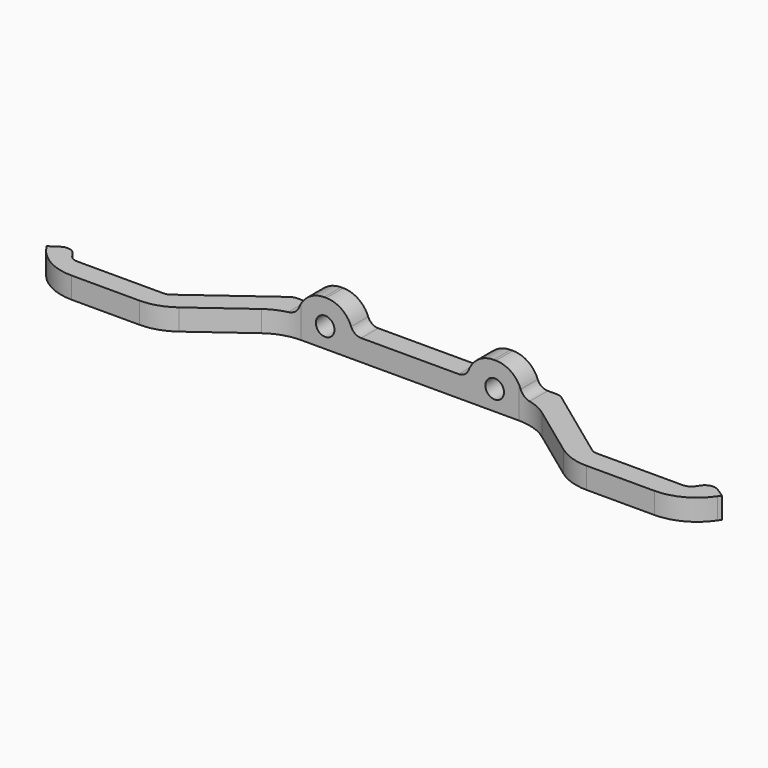
from build123d import *

# Parameters (mm, degrees)
F1_DEPTH    = 4
F2_W        = 9.5
F2_H        = 8.5
F3_DEPTH    = 4
F4_R        = 1.75
F5_DEPTH    = 154
F6_R        = 10
F7_R        = 2
F8_R        = 2
F9_T1_DEPTH = 26.6944612474
F9_T3_DEPTH = 26.6917420766


# Not quite as in the source:
# - a fillet or chamfer that OpenCascade refuses, or shapes differently, is made with other operations: its cross-section is extruded or revolved along the edge and cut away or added
# - an extrude ends at something that could not be found from the text; its depth is read off the source's solid


with BuildPart() as f1:
    # F0 (on Top) → F1 (new body)
    with BuildSketch(Plane.XY):
        Polygon((-82.859264966, -11), (-85, -7.7888974491), (-88.3282011774, -10.007698234), (-85, -15), (-63.6905180954, -15), (-48.6905180954, -4), (-1.3094819046, -4), (13.6905180954, -15), (35, -15), (38.3282011774, -10.007698234), (35, -7.7888974491), (32.859264966, -11), (15, -11), (0, 0), (-50, 0), (-65, -11), align=None)
    extrude(amount=F1_DEPTH)

    # F2 (on face) → F3 (join, through all)
    with BuildSketch(Plane(origin=(0, 0, 0), x_dir=(-1, 0, 0), z_dir=(0, 1, 0))):
        with Locations((9.1, 4.25)):
            Rectangle(F2_W, F2_H)
        with Locations((40.9, 4.25)):
            Rectangle(F2_W, F2_H)
    extrude(amount=-F3_DEPTH)

    # F4 (on face) → F5 (cut, through all)
    with BuildSketch(Plane(origin=(0, 0, 0), x_dir=(-1, 0, 0), z_dir=(0, 1, 0))):
        with Locations((9.1, 3.75)):
            Circle(F4_R)
        with Locations((40.9, 3.75)):
            Circle(F4_R)
    extrude(amount=-F5_DEPTH, mode=Mode.SUBTRACT)

    # F6
    f6_edges = [f1.edges().sort_by_distance(p)[0] for p in [
        (35, -15, 2),
        (13.690518, -15, 2),
        (-63.690518, -15, 2),
        (-85, -15, 2),
        (-48.690518, -4, 2),
        (-1.309482, -4, 2),
    ]]
    fillet(f6_edges, radius=F6_R)

    # F7
    f7_edges = [f1.edges().sort_by_distance(p)[0] for p in [
        (35, -7.788897, 2),
        (-85, -7.788897, 2),
        (-65, -11, 2),
        (-82.859265, -11, 2),
        (32.859265, -11, 2),
        (15, -11, 2),
        (0, 0, 2),
        (-50, 0, 2),
    ]]
    fillet(f7_edges, radius=F7_R)

    # F8
    f8_edges = [f1.edges().sort_by_distance(p)[0] for p in [
        (-45.65, -2.00136, 4),
        (-13.85, -2, 4),
        (-4.35, -2.00136, 4),
        (-36.15, -2, 4),
    ]]
    fillet(f8_edges, radius=F8_R)

    # F9: fillet of radius 5 on 4 edges, made by hand

    # F9_s2 → F9_t1 (cut)
    with BuildSketch(Plane.XZ.offset(-11.3458710383)):
        with BuildLine():
            ThreePointArc((-41.1116515847, 8.5), (-43.9463851322, 7.6187723552), (-45.7819004528, 5.2857142857))
            Line((-45.7819004528, 5.2857142857), (-46.2489253396, 5.4642857143))
            ThreePointArc((-46.2489253396, 5.4642857143), (-46.15, 6), (-46.15, 8.5))
            Line((-46.15, 8.5), (-45.65, 9))
            Line((-45.65, 9), (-41.1116515847, 9))
            Line((-41.1116515847, 9), (-41.1116515847, 8.5))
        make_face()
        with BuildLine():
            ThreePointArc((-4.2180995472, 5.2857142857), (-6.0536148677, 7.6187723552), (-8.8883484153, 8.5))
            Line((-8.8883484153, 8.5), (-8.8883484153, 9))
            Line((-8.8883484153, 9), (-4.35, 9))
            Line((-4.35, 9), (-3.85, 8.5))
            ThreePointArc((-3.85, 8.5), (-3.85, 6), (-3.7510746604, 5.4642857143))
            Line((-3.7510746604, 5.4642857143), (-4.2180995472, 5.2857142857))
        make_face()
    extrude(amount=F9_T1_DEPTH, mode=Mode.SUBTRACT)

    # F9_s4 → F9_t3 (cut)
    with BuildSketch(Plane.XZ.offset(-11.3458710383)):
        with BuildLine():
            ThreePointArc((-36.0180995472, 5.2857142857), (-37.8536148677, 7.6187723552), (-40.6883484153, 8.5))
            Line((-40.6883484153, 8.5), (-40.6883484153, 9))
            Line((-40.6883484153, 9), (-36.15, 9))
            Line((-36.15, 9), (-35.65, 8.5))
            ThreePointArc((-35.65, 8.5), (-35.65, 6), (-35.5510746604, 5.4642857143))
            Line((-35.5510746604, 5.4642857143), (-36.0180995472, 5.2857142857))
        make_face()
        with BuildLine():
            ThreePointArc((-9.3116515847, 8.5), (-12.1463851322, 7.6187723552), (-13.9819004528, 5.2857142857))
            Line((-13.9819004528, 5.2857142857), (-14.4489253396, 5.4642857143))
            ThreePointArc((-14.4489253396, 5.4642857143), (-14.35, 6), (-14.35, 8.5))
            Line((-14.35, 8.5), (-13.85, 9))
            Line((-13.85, 9), (-9.3116515847, 9))
            Line((-9.3116515847, 9), (-9.3116515847, 8.5))
        make_face()
    extrude(amount=F9_T3_DEPTH, mode=Mode.SUBTRACT)


solid = f1.part
